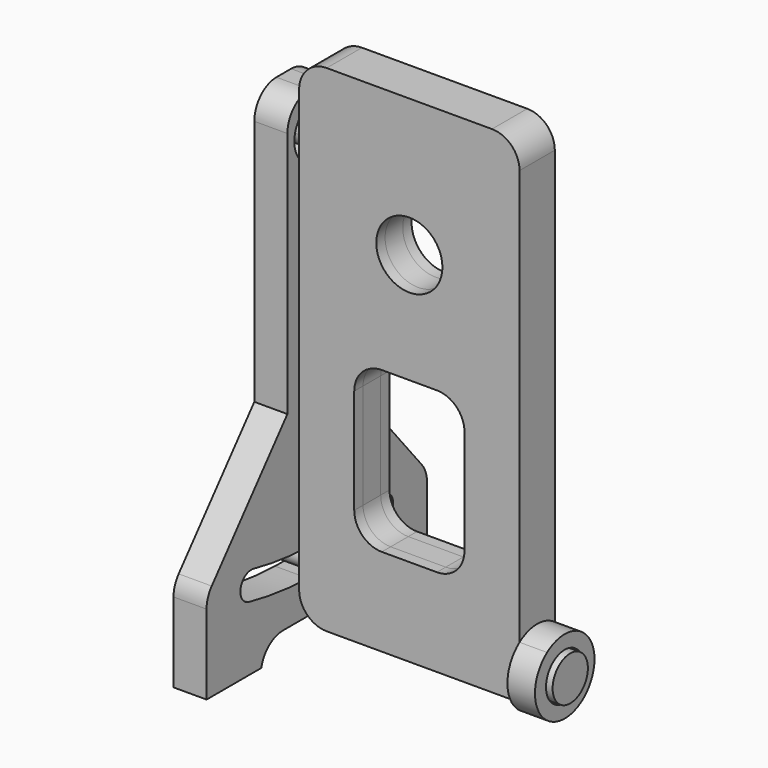
from build123d import *

# Parameters (mm, degrees)
F0_W           = 20
F0_H           = 29.0569514036
F0_R           = 6
F1_DEPTH       = 4
F3_DEPTH       = 8
F4_DEPTH       = 6
F5_DEPTH       = 8
F6_W           = 6
F6_H           = 12.9247409806
F6_H_2         = 12.42620707
F7_DEPTH       = 4
F8_R           = 5
F9_DEPTH       = 6
F10_T1_DEPTH   = 6
F10_T3_DEPTH   = 6
F10_T5_DEPTH   = 15.0823576644
F10_T7_DEPTH   = 31
F10_T9_DEPTH   = 30.9999999981
F10_T11_DEPTH  = 15.0353408704
F11_DEPTH      = 2
F11_DEPTH_BACK = 6
F13_DEPTH      = 6
F14_DEPTH      = 5


# Not quite as in the source:
# - a fillet or chamfer that OpenCascade refuses, or shapes differently, is made with other operations: its cross-section is extruded or revolved along the edge and cut away or added


with BuildPart() as f1:
    # F0 (on Front) → F1 (new body)
    with BuildSketch(Plane.XZ):
        Polygon((20, -45), (20, 45), (-20, 45), (-20, -45), (-10, -45), (10, -45), align=None)
        with Locations((0, -14.5284757018)):
            Rectangle(F0_W, F0_H, mode=Mode.SUBTRACT)
        with Locations((0, 20)):
            Circle(F0_R, mode=Mode.SUBTRACT)
    extrude(amount=F1_DEPTH)

    # F2 (on face) → F3 (join)
    with BuildSketch(Plane(origin=(-20, 0, 0), x_dir=(0, -1, 0), z_dir=(-1, 0, 0))):
        with BuildLine():
            Line((4, 29.8814751558), (4, 34.2185248442))
            ThreePointArc((4, 34.2185248442), (2, 35), (0, 34.2185248442))
            Line((0, 34.2185248442), (0, 29.8814751558))
            ThreePointArc((0, 29.8814751558), (2, 29.1), (4, 29.8814751558))
        make_face()
        with BuildLine():
            ThreePointArc((4.95, 32.05), (4.7020825302, 33.2337440602), (4, 34.2185248442))
            Line((4, 34.2185248442), (4, 29.8814751558))
            ThreePointArc((4, 29.8814751558), (4.7020825302, 30.8662559398), (4.95, 32.05))
        make_face()
        with BuildLine():
            Line((0, 29.8814751558), (0, 34.2185248442))
            ThreePointArc((0, 34.2185248442), (-0.95, 32.05), (0, 29.8814751558))
        make_face()
    extrude(amount=F3_DEPTH)

    # F2 (on face) → F5 (join)
    with BuildSketch(Plane(origin=(-20, 0, 0), x_dir=(0, -1, 0), z_dir=(-1, 0, 0))):
        with BuildLine():
            ThreePointArc((0, -36.5), (1.9999999971, -38.4999999971), (3.9999999942, -36.5))
            ThreePointArc((3.9999999942, -36.5), (1.9999999971, -34.5000000029), (0, -36.5))
        make_face()
    extrude(amount=F5_DEPTH)

    # F8
    f8_edges = [f1.edges().sort_by_distance(p)[0] for p in [
        (-20, -2, -45),
        (-10, -2, 0),
        (-10, -2, -29.056951),
        (10, -2, 0),
        (20, -2, 45),
        (-20, -2, 45),
        (10, -2, -29.056951),
    ]]
    fillet(f8_edges, radius=F8_R)

    # F11 (add, two sides): a face of the model
    f11_faces = [f1.faces().sort_by_distance(p)[0] for p in [
        (0.0348005991, -4, 1.935297002),
    ]]
    extrude(f11_faces, amount=F11_DEPTH)
    extrude(f11_faces, amount=-F11_DEPTH_BACK)

    # F12 (on face) → F13 (join)
    with BuildSketch(Plane.YZ.offset(20)):
        with BuildLine():
            ThreePointArc((-6, -40.8116131475), (-2.0000000273, -44.8116132021), (2, -40.8116132021))
            ThreePointArc((2, -40.8116132021), (-1.9999999727, -36.8116132021), (-6, -40.8116131475))
        make_face()
    extrude(amount=F13_DEPTH)


with BuildPart() as f4:
    # F2 (on face) → F4 (new body)
    with BuildSketch(Plane(origin=(-20, 0, 0), x_dir=(0, -1, 0), z_dir=(-1, 0, 0))):
        with BuildLine():
            ThreePointArc((4, 27.3585183577), (6.2549970623, 29.2384168161), (7.1, 32.05))
            ThreePointArc((7.1, 32.05), (6.2549970623, 34.8615831839), (4, 36.7414816423))
            Line((4, 36.7414816423), (4, 34.2185248442))
            ThreePointArc((4, 34.2185248442), (4.7020825302, 33.2337440602), (4.95, 32.05))
            ThreePointArc((4.95, 32.05), (4.7020825302, 30.8662559398), (4, 29.8814751558))
            Line((4, 29.8814751558), (4, 27.3585183577))
        make_face()
        with BuildLine():
            ThreePointArc((4, 36.7414816423), (6.2549970623, 34.8615831839), (7.1, 32.05))
            ThreePointArc((7.1, 32.05), (6.2549970623, 29.2384168161), (4, 27.3585183577))
            Line((4, 27.3585183577), (4, -33.9697129651))
            ThreePointArc((4, -33.9697129651), (10.1840030349, -33.4910145964), (16.2958364979, -32.4343512709))
            ThreePointArc((16.2958364979, -32.4343512709), (19.2776755505, -34.333992254), (17.3780345674, -37.3158313065))
            ThreePointArc((17.3780345674, -37.3158313065), (10.7283799691, -38.4618279661), (4, -38.9718452309))
            Line((4, -38.9718452309), (4, -45))
            Line((4, -45), (26.999999997, -45))
            Line((26.999999997, -45), (26.999999997, -32.7280576398))
            Line((26.999999997, -32.7280576398), (8.6701322833, -10.8303275913))
            Line((8.6701322833, -10.8303275913), (8.6701322833, 39))
            Line((8.6701322833, 39), (4, 39))
            Line((4, 39), (4, 36.7414816423))
        make_face()
        with BuildLine():
            Line((4, 34.2185248442), (4, 36.7414816423))
            ThreePointArc((4, 36.7414816423), (2, 37.15), (0, 36.7414816423))
            Line((0, 36.7414816423), (0, 34.2185248442))
            ThreePointArc((0, 34.2185248442), (2, 35), (4, 34.2185248442))
        make_face()
        with BuildLine():
            ThreePointArc((0, 36.7414816423), (2, 37.15), (4, 36.7414816423))
            Line((4, 36.7414816423), (4, 39))
            Line((4, 39), (0, 39))
            Line((0, 39), (0, 36.7414816423))
        make_face()
        with BuildLine():
            Line((4, -33.9697129651), (4, 27.3585183577))
            ThreePointArc((4, 27.3585183577), (2, 26.95), (0, 27.3585183577))
            Line((0, 27.3585183577), (0, -33.9697129651))
            ThreePointArc((0, -33.9697129651), (2, -34), (4, -33.9697129651))
        make_face()
        with BuildLine():
            ThreePointArc((0, 27.3585183577), (2, 26.95), (4, 27.3585183577))
            Line((4, 27.3585183577), (4, 29.8814751558))
            ThreePointArc((4, 29.8814751558), (2, 29.1), (0, 29.8814751558))
            Line((0, 29.8814751558), (0, 27.3585183577))
        make_face()
        with BuildLine():
            Line((0, 34.2185248442), (0, 36.7414816423))
            ThreePointArc((0, 36.7414816423), (-3.1, 32.05), (0, 27.3585183577))
            Line((0, 27.3585183577), (0, 29.8814751558))
            ThreePointArc((0, 29.8814751558), (-0.95, 32.05), (0, 34.2185248442))
        make_face()
        with BuildLine():
            ThreePointArc((0, 27.3585183577), (-3.1, 32.05), (0, 36.7414816423))
            Line((0, 36.7414816423), (0, 39))
            Line((0, 39), (-4.6701322773, 39))
            Line((-4.6701322773, 39), (-4.6701322811, -10.6818171995))
            Line((-4.6701322811, -10.6818171995), (-23.000000003, -32.7280576398))
            Line((-23.000000003, -32.7280576398), (-23.000000003, -45))
            Line((-23.000000003, -45), (0, -45))
            Line((0, -45), (0, -38.9718452309))
            ThreePointArc((0, -38.9718452309), (-6.7283799721, -38.4618279657), (-13.3780345732, -37.3158313052))
            ThreePointArc((-13.3780345732, -37.3158313052), (-15.2776755561, -34.3339922525), (-12.2958365033, -32.4343512697))
            ThreePointArc((-12.2958365033, -32.4343512697), (-6.1840030376, -33.4910145961), (0, -33.9697129651))
            Line((0, -33.9697129651), (0, 27.3585183577))
        make_face()
        with BuildLine():
            Line((4, -45), (4, -38.9718452309))
            ThreePointArc((4, -38.9718452309), (2, -39), (0, -38.9718452309))
            Line((0, -38.9718452309), (0, -45))
            Line((0, -45), (4, -45))
        make_face()
    extrude(amount=F4_DEPTH)

    # F6 (on face) → F7 (join)
    with BuildSketch(Plane(origin=(0, 0, -45), x_dir=(1, 0, 0), z_dir=(0, 0, -1))):
        with Locations((-23, -16.5376295127)):
            Rectangle(F6_W, F6_H)
        with Locations((-23, 20.786896462)):
            Rectangle(F6_W, F6_H_2)
    extrude(amount=F7_DEPTH)

    # F2 (on face) → F9 (cut, through all)
    with BuildSketch(Plane(origin=(-20, 0, 0), x_dir=(0, -1, 0), z_dir=(-1, 0, 0))):
        with BuildLine():
            Line((4, 34.2185248442), (4, 36.7414816423))
            ThreePointArc((4, 36.7414816423), (2, 37.15), (0, 36.7414816423))
            Line((0, 36.7414816423), (0, 34.2185248442))
            ThreePointArc((0, 34.2185248442), (2, 35), (4, 34.2185248442))
        make_face()
        with BuildLine():
            Line((0, 34.2185248442), (0, 36.7414816423))
            ThreePointArc((0, 36.7414816423), (-3.1, 32.05), (0, 27.3585183577))
            Line((0, 27.3585183577), (0, 29.8814751558))
            ThreePointArc((0, 29.8814751558), (-0.95, 32.05), (0, 34.2185248442))
        make_face()
        with BuildLine():
            ThreePointArc((0, 27.3585183577), (2, 26.95), (4, 27.3585183577))
            Line((4, 27.3585183577), (4, 29.8814751558))
            ThreePointArc((4, 29.8814751558), (2, 29.1), (0, 29.8814751558))
            Line((0, 29.8814751558), (0, 27.3585183577))
        make_face()
        with BuildLine():
            ThreePointArc((4, 27.3585183577), (6.2549970623, 29.2384168161), (7.1, 32.05))
            ThreePointArc((7.1, 32.05), (6.2549970623, 34.8615831839), (4, 36.7414816423))
            Line((4, 36.7414816423), (4, 34.2185248442))
            ThreePointArc((4, 34.2185248442), (4.7020825302, 33.2337440602), (4.95, 32.05))
            ThreePointArc((4.95, 32.05), (4.7020825302, 30.8662559398), (4, 29.8814751558))
            Line((4, 29.8814751558), (4, 27.3585183577))
        make_face()
    extrude(amount=F9_DEPTH, mode=Mode.SUBTRACT)

    # F10: fillet of radius 5 on 6 edges, made by hand

    # F10_s2 → F10_t1 (join)
    with BuildSketch(Plane.YZ.offset(-26)):
        with BuildLine():
            ThreePointArc((-14.573792927, -49), (-12.8370911016, -46.1270166538), (-9.6748134414, -45))
            Line((-9.6748134414, -45), (-14.573792927, -45))
            Line((-14.573792927, -45), (-14.573792927, -49))
        make_face()
    extrude(amount=F10_T1_DEPTH)

    # F10_s4 → F10_t3 (join)
    with BuildSketch(Plane.YZ.offset(-26)):
        with BuildLine():
            ThreePointArc((5.1762795368, -45), (8.338557197, -46.1270166538), (10.0752590224, -49))
            Line((10.0752590224, -49), (10.0752590224, -45))
            Line((10.0752590224, -45), (5.1762795368, -45))
        make_face()
    extrude(amount=F10_T3_DEPTH)

    # F10_s6 → F10_t5 (cut)
    with BuildSketch(Plane.YZ.offset(-30.5411788322)):
        with BuildLine():
            ThreePointArc((-26.999999997, -34.5445291727), (-26.6994831746, -32.8372336905), (-25.8340568515, -31.3351666135))
            Line((-25.8340568515, -31.3351666135), (-26.999999997, -32.7280576398))
            Line((-26.999999997, -32.7280576398), (-26.999999997, -34.5445291727))
        make_face()
    extrude(amount=F10_T5_DEPTH, mode=Mode.SUBTRACT)

    # F10_s8 → F10_t7 (cut)
    with BuildSketch(Plane.YZ.offset(-38.5)):
        with BuildLine():
            ThreePointArc((-3.6701322833, 39), (-7.2056661892, 37.5355339059), (-8.6701322833, 34))
            Line((-8.6701322833, 34), (-8.6701322833, 39))
            Line((-8.6701322833, 39), (-3.6701322833, 39))
        make_face()
    extrude(amount=F10_T7_DEPTH, mode=Mode.SUBTRACT)

    # F10_s10 → F10_t9 (cut)
    with BuildSketch(Plane.YZ.offset(-38.499999999)):
        with BuildLine():
            ThreePointArc((4.6701322777, 34.0000000004), (3.2056661835, 37.5355339061), (-0.3298677223, 39))
            Line((-0.3298677223, 39), (4.6701322773, 39))
            Line((4.6701322773, 39), (4.6701322777, 34.0000000004))
        make_face()
    extrude(amount=F10_T9_DEPTH, mode=Mode.SUBTRACT)

    # F10_s12 → F10_t11 (cut)
    with BuildSketch(Plane.YZ.offset(-30.5176704352)):
        with BuildLine():
            ThreePointArc((23.000000003, -34.5351258139), (22.7023148902, -32.8356450985), (21.8447061222, -31.3385284265))
            Line((21.8447061222, -31.3385284265), (23.000000003, -32.7280576398))
            Line((23.000000003, -32.7280576398), (23.000000003, -34.5351258139))
        make_face()
    extrude(amount=F10_T11_DEPTH, mode=Mode.SUBTRACT)


with BuildPart() as f14:
    # F12 (on face) → F14 (new body)
    with BuildSketch(Plane.YZ.offset(20)):
        with BuildLine():
            Line((2, -45), (2, -42.2477538637))
            ThreePointArc((2, -42.2477538637), (0.7323612075, -44.0668708312), (-1.2789479692, -45))
            Line((-1.2789479692, -45), (0, -45))
            Line((0, -45), (2, -45))
        make_face()
        with BuildLine():
            ThreePointArc((2.25, -40.8116132021), (2.1870335561, -41.540482189), (2, -42.2477538637))
            Line((2, -42.2477538637), (2, -45))
            Line((2, -45), (0, -45))
            Line((0, -45), (-1.2789479692, -45))
            ThreePointArc((-1.2789479692, -45), (-2, -45.0616132021), (-2.7210520308, -45))
            Line((-2.7210520308, -45), (-4, -45))
            Line((-4, -45), (-6, -45))
            Line((-6, -45), (-6, -42.2477538637))
            ThreePointArc((-6, -42.2477538637), (-6.25, -40.8116132021), (-6, -39.3754725405))
            Line((-6, -39.3754725405), (-6, -35.3744724094))
            ThreePointArc((-6, -35.3744724094), (-5.0465144017, -46.8350051037), (4.75, -40.8116132021))
            ThreePointArc((4.75, -40.8116132021), (4.0233919016, -37.7650988004), (2, -35.3744724094))
            Line((2, -35.3744724094), (2, -39.3754725405))
            ThreePointArc((2, -39.3754725405), (2.1870335561, -40.0827442152), (2.25, -40.8116132021))
        make_face()
        with BuildLine():
            ThreePointArc((-6, -39.3754725405), (-2, -36.5616132021), (2, -39.3754725405))
            Line((2, -39.3754725405), (2, -35.3744724094))
            ThreePointArc((2, -35.3744724094), (-2, -34.0616132021), (-6, -35.3744724094))
            Line((-6, -35.3744724094), (-6, -39.3754725405))
        make_face()
        with BuildLine():
            ThreePointArc((-2.7210520308, -45), (-4.7323612075, -44.0668708312), (-6, -42.2477538637))
            Line((-6, -42.2477538637), (-6, -45))
            Line((-6, -45), (-4, -45))
            Line((-4, -45), (-2.7210520308, -45))
        make_face()
    extrude(amount=F14_DEPTH)


solid = Compound([f1.part, f4.part, f14.part])
